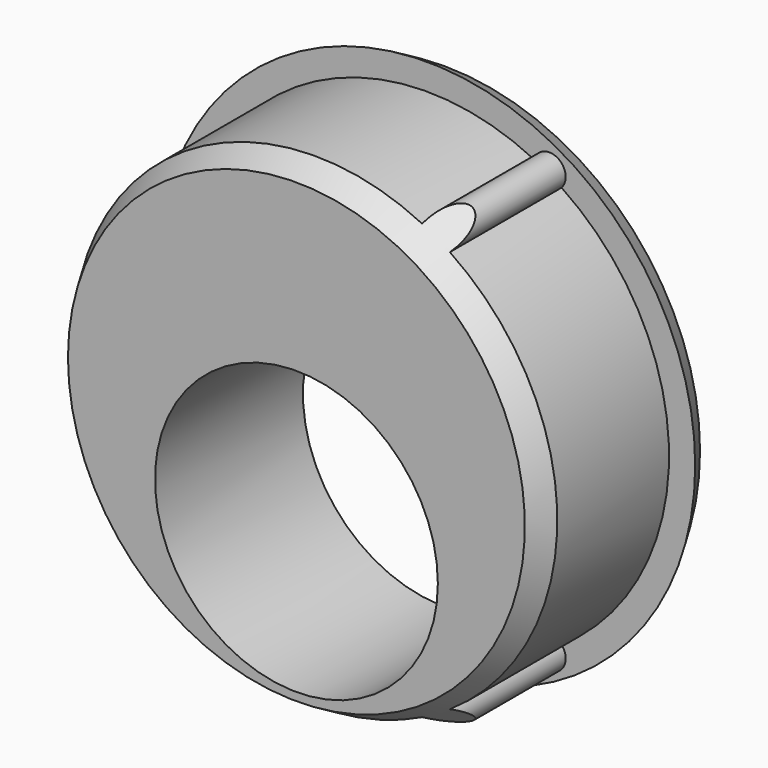
from build123d import *

# Parameters (mm, degrees)
F0_R          = 22.25
F0_R_2        = 13
F1_DEPTH      = 15
F1_DEPTH_BACK = 2
F4_R          = 1.5
F5_DEPTH      = 15


with BuildPart() as f1:
    # F0 (on Front) → F1 (new body, two sides)
    with BuildSketch(Plane.XZ) as f1_sk:
        Circle(F0_R)
        with Locations((0, -7.25)):
            Circle(F0_R_2, mode=Mode.SUBTRACT)
    extrude(amount=F1_DEPTH)
    extrude(f1_sk.sketch, amount=-F1_DEPTH_BACK)

    # F2 (on Top) → F3 (revolve)
    with BuildSketch(Plane.XY):
        Polygon((-24.6547005384, 0), (-21.5, 0), (-21.5, 2), (-23.5, 2), align=None)
    revolve(axis=Axis((0, 0, 0), (0, 1, 0)))

    # F4 (on Front) → F5 (join, through all)
    with BuildSketch(Plane.XZ):
        with Locations((-22.5, 0)):
            Circle(F4_R)
        with Locations((11.25, -19.4855715851)):
            Circle(F4_R)
        with Locations((11.25, 19.4855715851)):
            Circle(F4_R)
    extrude(amount=F5_DEPTH)

    # F6 (on Top) → F7 (revolve, cut)
    with BuildSketch(Plane.XY):
        Polygon((-24.8129580218, -15), (-21, -15), (-24.8129580218, -8.3957629791), align=None)
    revolve(axis=Axis((0, 0, 0), (0, 1, 0)), mode=Mode.SUBTRACT)


solid = f1.part
